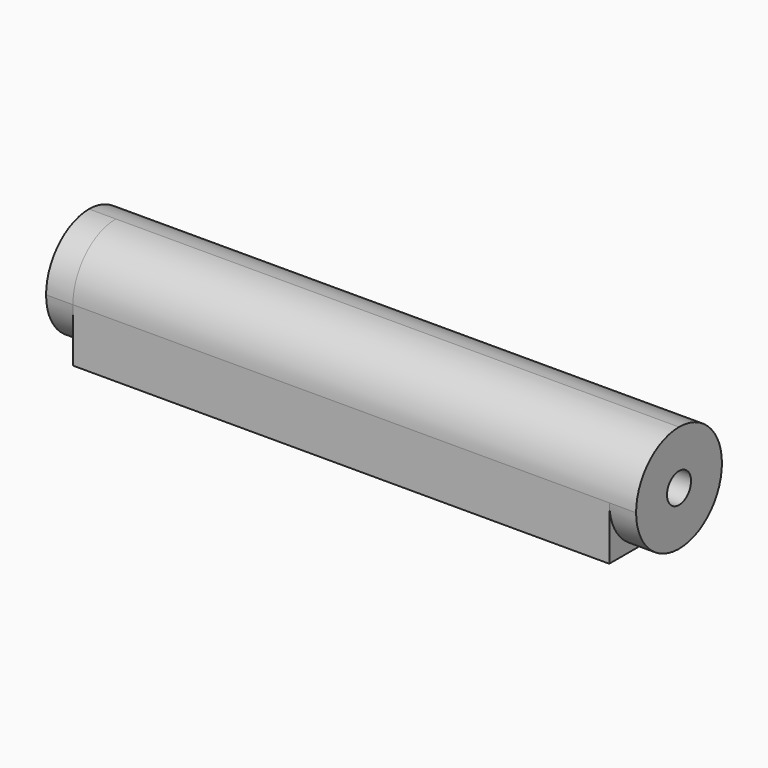
from build123d import *

# Parameters (mm, degrees)
F0_W      = 55
F0_H      = 10
F1_DEPTH  = 10
F3_D      = 2.8
F3_DEPTH  = 13
F3_TIP    = 0.8412048666
F5_D      = 2.8
F5_DEPTH  = 13
F5_TIP    = 0.8412048666
F7_DEPTH  = 2.5
F9_DEPTH  = 2.5
F10_R     = 4.9999
F12_D     = 1.8
F12_DEPTH = 5
F12_TIP   = 0.5407745571


# Not quite as in the source:
# - a fillet or chamfer is up to 0.001 mm smaller than in the source, because OpenCascade refuses the exact size
# - a feature names something its author has since deleted; it is built from what else it names


with BuildPart() as f1:
    # F0 (on Top) → F1 (new body)
    with BuildSketch(Plane.XY):
        Rectangle(F0_W, F0_H)
    extrude(amount=F1_DEPTH)

    # F3
    with Locations(Plane(origin=(-27.5, 0, 0), x_dir=(0, -1, 0), z_dir=(-1, 0, 0))):
        with Locations((0, 5)):
            Hole(F3_D / 2, depth=F3_DEPTH)
            with Locations((0, 0, -(F3_DEPTH + F3_TIP / 2))):  # 118° drill point
                Cone(0, F3_D / 2, F3_TIP, mode=Mode.SUBTRACT)

    # F5
    with Locations(Plane.YZ.offset(27.5)):
        with Locations((0, 5)):
            Hole(F5_D / 2, depth=F5_DEPTH)
            with Locations((0, 0, -(F5_DEPTH + F5_TIP / 2))):  # 118° drill point
                Cone(0, F5_D / 2, F5_TIP, mode=Mode.SUBTRACT)

    # F6 (on face) → F7 (cut)
    with BuildSketch(Plane.YZ.offset(27.5)):
        with BuildLine():
            Line((5, 0), (5, 5))
            ThreePointArc((5, 5), (3.5355339059, 1.4644660941), (0, 0))
            Line((0, 0), (5, 0))
        make_face()
        with BuildLine():
            Line((-5, 0), (0, 0))
            ThreePointArc((0, 0), (-3.5355339059, 1.4644660941), (-5, 5))
            Line((-5, 5), (-5, 0))
        make_face()
    extrude(amount=-F7_DEPTH, mode=Mode.SUBTRACT)

    # F8 (on face) → F9 (cut)
    with BuildSketch(Plane(origin=(-27.5, 0, 0), x_dir=(0, -1, 0), z_dir=(-1, 0, 0))):
        with BuildLine():
            Line((5, 0), (5, 5))
            ThreePointArc((5, 5), (3.5355339059, 1.4644660941), (0, 0))
            Line((0, 0), (5, 0))
        make_face()
        with BuildLine():
            ThreePointArc((0, 10), (3.5355339059, 8.5355339059), (5, 5))
            Line((5, 5), (5, 10))
            Line((5, 10), (0, 10))
        make_face()
        with BuildLine():
            Line((-5, 0), (0, 0))
            ThreePointArc((0, 0), (-3.5355339059, 1.4644660941), (-5, 5))
            Line((-5, 5), (-5, 0))
        make_face()
    extrude(amount=-F9_DEPTH, mode=Mode.SUBTRACT)

    # F10 (radius 5 in the source; OpenCascade refuses exactly that, so slightly less here)
    f10_edges = [f1.edges().sort_by_distance(p)[0] for p in [
        (0, 5, 10),
        (1.25, -5, 10),
    ]]
    fillet(f10_edges, radius=F10_R)

    # F12
    with Locations(Plane(origin=(0, 0, 0), x_dir=(1, 0, 0), z_dir=(0, 0, -1))):
        with Locations((-20, 0), (20, 0)):
            Hole(F12_D / 2, depth=F12_DEPTH)
            with Locations((0, 0, -(F12_DEPTH + F12_TIP / 2))):  # 118° drill point
                Cone(0, F12_D / 2, F12_TIP, mode=Mode.SUBTRACT)


solid = f1.part
